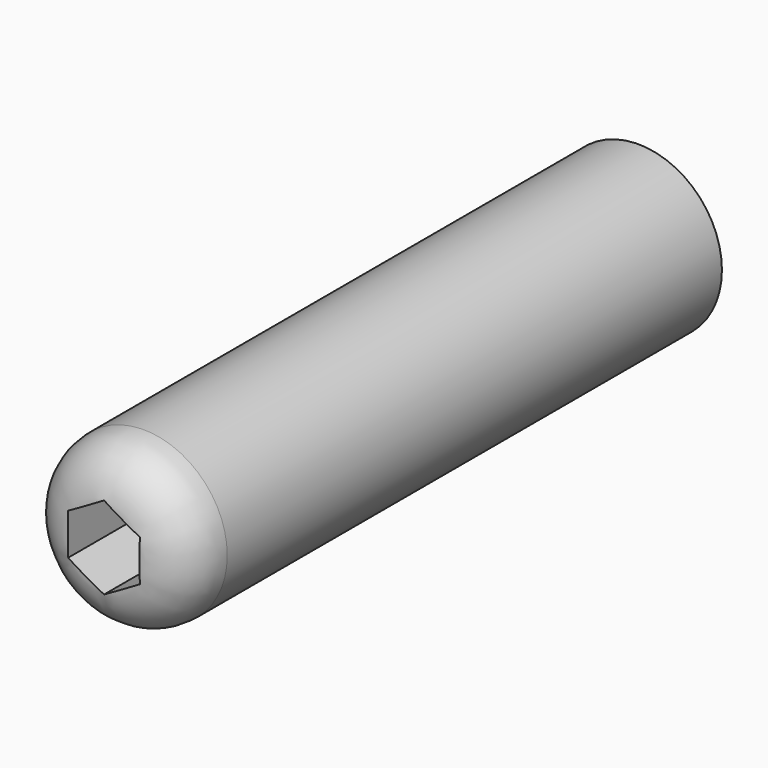
from build123d import *

# Parameters (mm, degrees)
F0_R     = 2.032
F1_DEPTH = 6.35
F0_R_2   = 12.7
F2_DEPTH = 101.6


# Not quite as in the source:
# - a fillet or chamfer that OpenCascade refuses, or shapes differently, is made with other operations: its cross-section is extruded or revolved along the edge and cut away or added
# - the program builds the solid bodies; features that only make, move or delete a surface that nothing else refers to are left out


with BuildPart() as f1:
    # F0 (on Front) → F1 (new body)
    with BuildSketch(Plane.XZ):
        Polygon((-5.4516299168, -3.1475), (0, -6.295), (5.4516299168, -3.1475), (5.4516299168, 3.1475), (0, 6.295), (-5.4516299168, 3.1475), align=None)
        Circle(F0_R, mode=Mode.SUBTRACT)
    extrude(amount=F1_DEPTH)

    # F0 (on Front) → F2 (join)
    with BuildSketch(Plane.XZ):
        Circle(F0_R_2)
        Polygon((5.4516299168, -3.1475), (0, -6.295), (-5.4516299168, -3.1475), (-5.4516299168, 3.1475), (0, 6.295), (5.4516299168, 3.1475), align=None, mode=Mode.SUBTRACT)
    extrude(amount=F2_DEPTH)

    # F3: fillet of radius 7.62 on 1 edges, made by hand

    # F3_s1 → F3_t2 (revolve, cut)
    with BuildSketch(Plane.XY):
        with BuildLine():
            ThreePointArc((12.7, -93.98), (10.4681536726, -99.3681536726), (5.08, -101.6))
            Line((5.08, -101.6), (12.7, -101.6))
            Line((12.7, -101.6), (12.7, -93.98))
        make_face()
    revolve(axis=Axis((0, -101.6, 0), (0, -1, 0)), mode=Mode.SUBTRACT)


solid = f1.part
